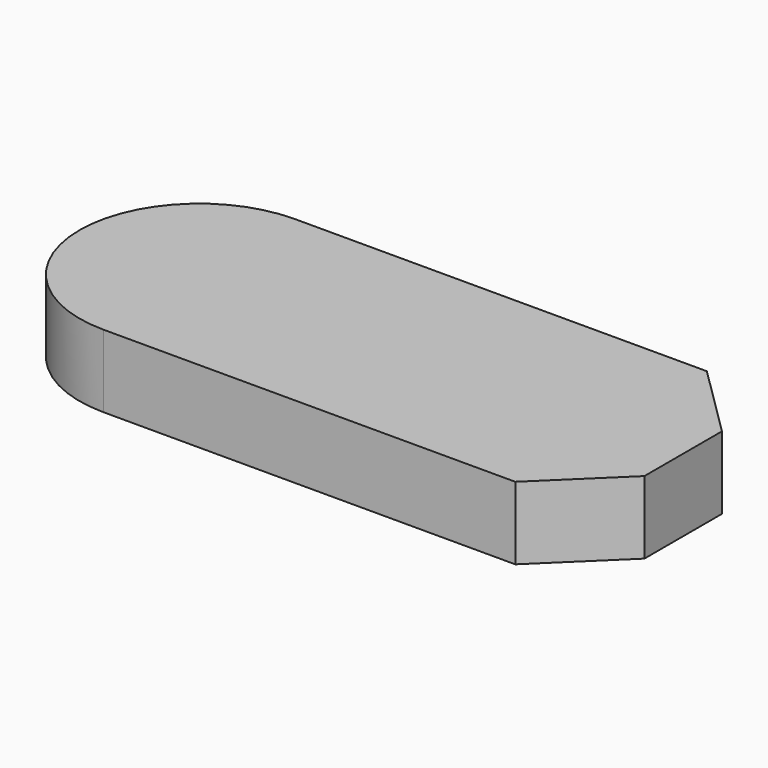
from build123d import *

# Parameters (mm, degrees)
F0_W     = 18
F0_H     = 29.6524400212
F1_DEPTH = 9


# Not quite as in the source:
# - a feature names something its author has since deleted; it is built from what else it names


with BuildPart() as f1:
    # F0 (on Top) → F1 (new body)
    with BuildSketch(Plane.XY):
        with Locations((9, 14.8262200106)):
            Rectangle(F0_W, F0_H)
        with BuildLine():
            ThreePointArc((0, 29.6524400212), (-14.8262200106, 14.8262200106), (0, 0))
            Line((0, 0), (0, 29.6524400212))
        make_face()
        Polygon((18, 29.6524400212), (18, 0), (51, 0), (60, 8.7334750722), (60, 20.7334750722), (51, 29.6524400212), align=None)
    extrude(amount=F1_DEPTH)


solid = f1.part
